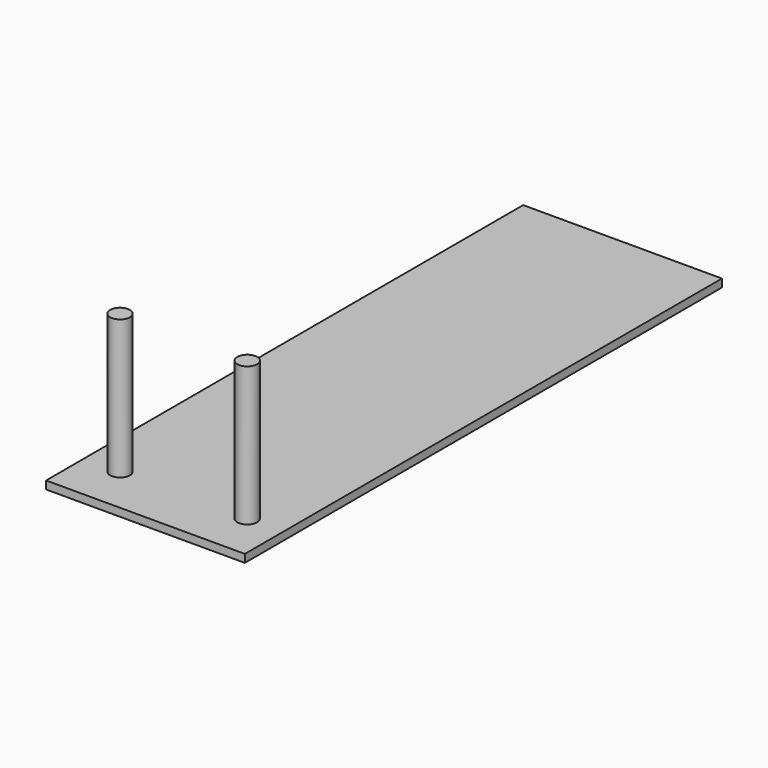
from build123d import *

# Parameters (mm, degrees)
F0_W     = 50
F0_H     = 150
F1_DEPTH = 2
F2_R     = 2.5
F3_DEPTH = 35


# Not quite as in the source:
# - a pattern or mirror of a feature is missing from the dataset's text; its kind, count and spacing are read off the source's solid


with BuildPart() as f1:
    # F0 (on Top) → F1 (new body)
    with BuildSketch(Plane.XY):
        Rectangle(F0_W, F0_H)
    extrude(amount=F1_DEPTH)

    # F2 (on face) → F3 (join)
    with BuildSketch(Plane.XY.offset(2)):
        with Locations((-16, -63)):
            Circle(F2_R)
    f3 = extrude(amount=F3_DEPTH)

    # F3_copies: F3 across plane
    add(f3.mirror(Plane(origin=(0, 0, 0), x_dir=(0, 0, 1), z_dir=(1, 0, 0))))


solid = f1.part
